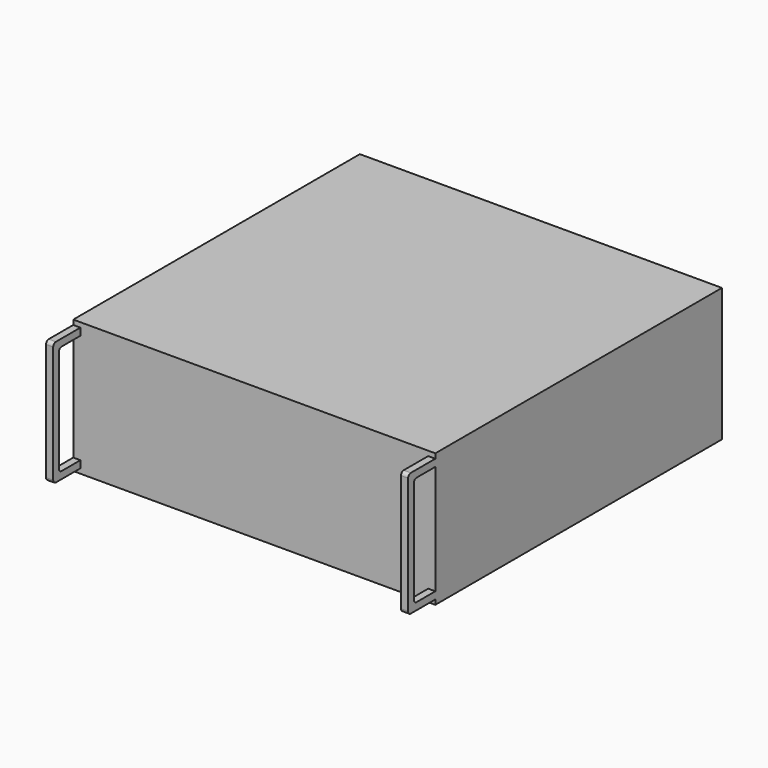
from build123d import *

# Parameters (mm, degrees)
F0_W     = 482.6
F0_H     = 177.8
F1_DEPTH = 477.52
F4_DEPTH = 9.525
F5_R     = 4.445


# Not quite as in the source:
# - a pattern or mirror of a feature is missing from the dataset's text; its kind, count and spacing are read off the source's solid


with BuildPart() as f1:
    # F0 (on Front) → F1 (new body)
    with BuildSketch(Plane.XZ):
        Rectangle(F0_W, F0_H)
    extrude(amount=-F1_DEPTH)

    # F3 (on offset) → F4 (join)
    with BuildSketch(Plane.YZ.offset(241.3)):
        Polygon((0, 73.025), (0, 82.55), (-45.2747344971, 82.55), (-45.2747344971, -82.55), (0, -82.55), (0, -73.025), (-35.7497344971, -73.025), (-35.7497344971, 73.025), align=None)
    f4 = extrude(amount=-F4_DEPTH)

    # F4_copies: F4 across plane
    add(f4.mirror(Plane(origin=(0, 0, 0), x_dir=(0, 0, -1), z_dir=(-1, 0, 0))))

    # F5
    f5_edges = [f1.edges().sort_by_distance(p)[0] for p in [
        (236.5375, -45.274734, 82.55),
        (236.5375, -45.274734, -82.55),
        (236.5375, -35.749734, -73.025),
        (236.5375, -35.749734, 73.025),
        (-236.5375, -45.274734, -82.55),
        (-236.5375, -35.749734, -73.025),
        (-236.5375, -35.749734, 73.025),
        (-236.5375, -45.274734, 82.55),
    ]]
    fillet(f5_edges, radius=F5_R)


solid = f1.part
